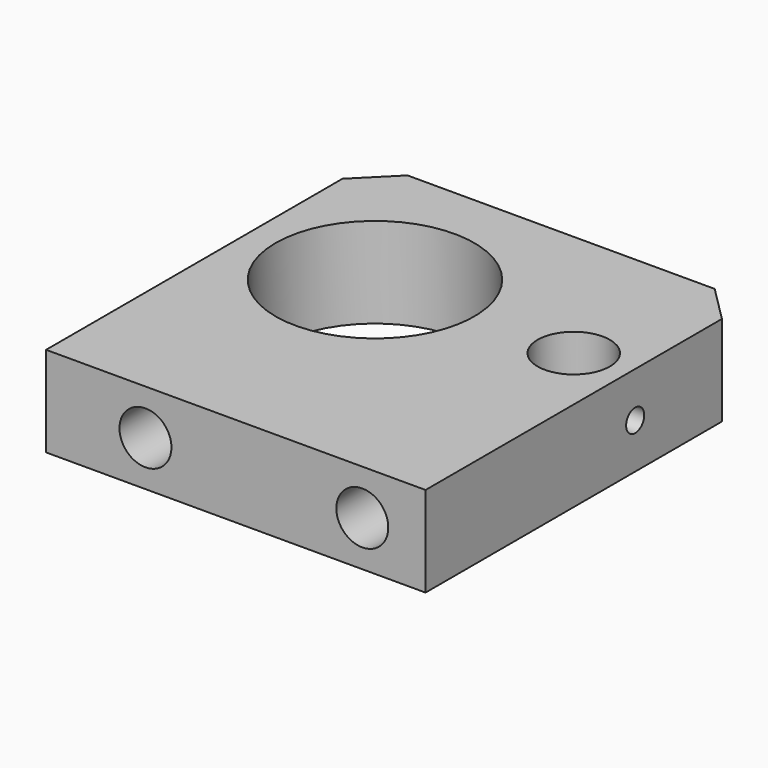
from build123d import *

# Parameters (mm, degrees)
F1_DEPTH = 10
F3_D     = 22
F4_D     = 8
F6_D     = 2.5
F6_DEPTH = 5
F6_TIP   = 0.7510757738
F8_D     = 5.75
F8_DEPTH = 11
F8_TIP   = 1.7274742797


# Not quite as in the source:
# - a feature names something its author has since deleted; it is built from what else it names


with BuildPart() as f1:
    # F0 (on Top) → F1 (new body)
    with BuildSketch(Plane.XY):
        Polygon((-6.5280715935, -6.1914156973), (-6.5280715935, -47.1914156973), (35.4719284065, -47.1914156973), (35.4719284065, -6.1914156973), (31.4719284065, -2.1914156973), (-2.5280715935, -2.1914156973), align=None)
    extrude(amount=F1_DEPTH)

    # F3 (through all)
    with Locations(Plane.XY.offset(10)):
        with Locations((7.4719284065, -19.1914156973)):
            Hole(F3_D / 2)

    # F4 (through all)
    with Locations(Plane.XY.offset(10)):
        with Locations((29.4719284065, -19.1914156973)):
            Hole(F4_D / 2)

    # F6
    with Locations(Plane.YZ.offset(35.4719284065)):
        with Locations((-18.1914156973, 5)):
            Hole(F6_D / 2, depth=F6_DEPTH)
            with Locations((0, 0, -(F6_DEPTH + F6_TIP / 2))):  # 118° drill point
                Cone(0, F6_D / 2, F6_TIP, mode=Mode.SUBTRACT)

    # F8
    with Locations(Plane.XZ.offset(47.1914156973)):
        with Locations((28.4719284065, 5), (4.4719284065, 5)):
            Hole(F8_D / 2, depth=F8_DEPTH)
            with Locations((0, 0, -(F8_DEPTH + F8_TIP / 2))):  # 118° drill point
                Cone(0, F8_D / 2, F8_TIP, mode=Mode.SUBTRACT)


solid = f1.part
